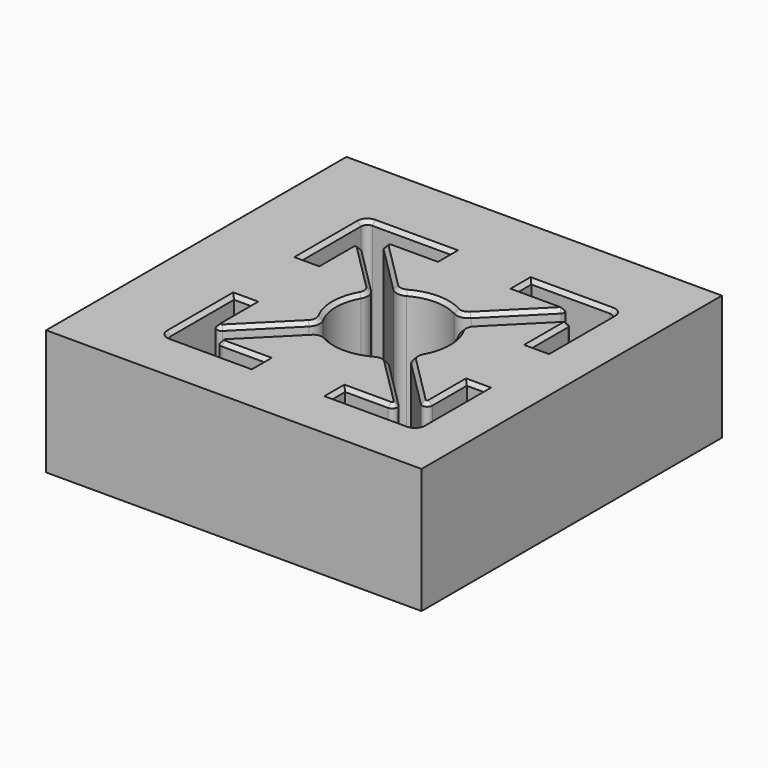
from build123d import *

# Parameters (mm, degrees)
F0_W     = 30
F0_H     = 30
F1_DEPTH = 10
F2_SIZE  = 0.29999


# Not quite as in the source:
# - a fillet or chamfer is up to 0.001 mm smaller than in the source, because OpenCascade refuses the exact size


with BuildPart() as f1:
    # F0 (on Top) → F1 (new body)
    with BuildSketch(Plane.XY):
        with Locations((8.7794362941, 10.8101805312)):
            Rectangle(F0_W, F0_H)
        with BuildLine():
            Line((13.2, 20), (19.5, 20))
            ThreePointArc((19.5, 20), (19.8535533906, 19.8535533906), (20, 19.5))
            Line((20, 19.5), (20, 13.2))
            Line((20, 13.2), (18.6, 13.2))
            Line((18.6, 13.2), (18.6, 16.8857864376))
            ThreePointArc((18.6, 16.8857864376), (18.4148050297, 17.1629502974), (18.0878679656, 17.097918472))
            Line((18.0878679656, 17.097918472), (14.0849274668, 13.0949779732))
            ThreePointArc((14.0849274668, 13.0949779732), (13.8016579584, 12.5262720767), (13.918171677, 11.9016981704))
            ThreePointArc((13.918171677, 11.9016981704), (14.4115666356, 10), (13.918171677, 8.0983018296))
            ThreePointArc((13.918171677, 8.0983018296), (13.8016579584, 7.4737279233), (14.0849274668, 6.9050220268))
            Line((14.0849274668, 6.9050220268), (17.9171572875, 3.0727922061))
            ThreePointArc((17.9171572875, 3.0727922061), (18.3530733729, 2.9860831056), (18.6, 3.3556349186))
            Line((18.6, 3.3556349186), (18.6, 6.8))
            Line((18.6, 6.8), (20, 6.8))
            Line((20, 6.8), (20, 0.5))
            ThreePointArc((20, 0.5), (19.8535533906, 0.1464466094), (19.5, 0))
            Line((19.5, 0), (13.2, 0))
            Line((13.2, 0), (13.2, 1.4))
            Line((13.2, 1.4), (16.6443650814, 1.4))
            ThreePointArc((16.6443650814, 1.4), (17.0139168944, 1.6469266271), (16.9272077939, 2.0828427125))
            Line((16.9272077939, 2.0828427125), (13.0949779732, 5.9150725332))
            ThreePointArc((13.0949779732, 5.9150725332), (12.5262720767, 6.1983420416), (11.9016981704, 6.081828323))
            ThreePointArc((11.9016981704, 6.081828323), (10, 5.5884333644), (8.0983018296, 6.081828323))
            ThreePointArc((8.0983018296, 6.081828323), (7.4737279233, 6.1983420416), (6.9050220268, 5.9150725332))
            Line((6.9050220268, 5.9150725332), (3.0727922061, 2.0828427125))
            ThreePointArc((3.0727922061, 2.0828427125), (2.9860831056, 1.6469266271), (3.3556349186, 1.4))
            Line((3.3556349186, 1.4), (6.8, 1.4))
            Line((6.8, 1.4), (6.8, 0))
            Line((6.8, 0), (0.5, 0))
            ThreePointArc((0.5, 0), (0.1464466094, 0.1464466094), (0, 0.5))
            Line((0, 0.5), (0, 6.8))
            Line((0, 6.8), (1.4, 6.8))
            Line((1.4, 6.8), (1.4, 3.3556349186))
            ThreePointArc((1.4, 3.3556349186), (1.6469266271, 2.9860831056), (2.0828427125, 3.0727922061))
            Line((2.0828427125, 3.0727922061), (5.9150725332, 6.9050220268))
            ThreePointArc((5.9150725332, 6.9050220268), (6.1983420416, 7.4737279233), (6.081828323, 8.0983018296))
            ThreePointArc((6.081828323, 8.0983018296), (5.5884333644, 10), (6.081828323, 11.9016981704))
            ThreePointArc((6.081828323, 11.9016981704), (6.1983420416, 12.5262720767), (5.9150725332, 13.0949779732))
            Line((5.9150725332, 13.0949779732), (2.0828427125, 16.9272077939))
            ThreePointArc((2.0828427125, 16.9272077939), (1.6469266271, 17.0139168944), (1.4, 16.6443650814))
            Line((1.4, 16.6443650814), (1.4, 13.2))
            Line((1.4, 13.2), (0, 13.2))
            Line((0, 13.2), (0, 19.5))
            ThreePointArc((0, 19.5), (0.1464466094, 19.8535533906), (0.5, 20))
            Line((0.5, 20), (6.8, 20))
            Line((6.8, 20), (6.8, 18.6))
            Line((6.8, 18.6), (3.3556349186, 18.6))
            ThreePointArc((3.3556349186, 18.6), (2.9860831056, 18.3530733729), (3.0727922061, 17.9171572875))
            Line((3.0727922061, 17.9171572875), (6.9050220268, 14.0849274668))
            ThreePointArc((6.9050220268, 14.0849274668), (7.4737279233, 13.8016579584), (8.0983018296, 13.918171677))
            ThreePointArc((8.0983018296, 13.918171677), (10, 14.4115666356), (11.9016981704, 13.918171677))
            ThreePointArc((11.9016981704, 13.918171677), (12.5262720767, 13.8016579584), (13.0949779732, 14.0849274668))
            Line((13.0949779732, 14.0849274668), (17.097918472, 18.0878679656))
            ThreePointArc((17.097918472, 18.0878679656), (17.1629502974, 18.4148050297), (16.8857864376, 18.6))
            Line((16.8857864376, 18.6), (13.2, 18.6))
            Line((13.2, 18.6), (13.2, 20))
        make_face(mode=Mode.SUBTRACT)
    extrude(amount=F1_DEPTH)

    # F2 (size 0.3 in the source; OpenCascade refuses exactly that, so slightly less here)
    f2_edges = [f1.edges().sort_by_distance(p)[0] for p in [
        (0, 16.35, 10),
        (4.988907, 16.001042, 10),
        (3.998958, 15.011093, 10),
        (7.473728, 6.198342, 10),
        (14.411567, 10, 10),
        (19.3, 13.2, 10),
        (16.35, 20, 10),
        (13.2, 19.3, 10),
        (6.8, 19.3, 10),
        (20, 3.65, 10),
        (13.2, 0.7, 10),
        (6.8, 0.7, 10),
        (0.7, 6.8, 10),
        (19.3, 6.8, 10),
        (0, 3.65, 10),
    ]]
    chamfer(f2_edges, length=F2_SIZE)


solid = f1.part
